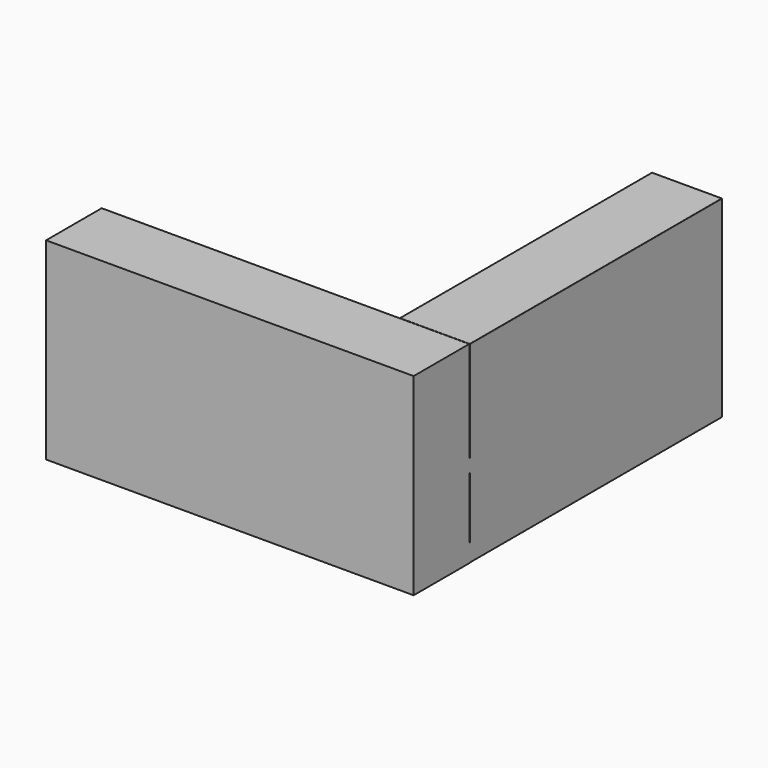
from build123d import *

# Parameters (mm, degrees)
F1_DEPTH = 1800
F3_DEPTH = 1800
F4_DEPTH = 1800
F6_DEPTH = 2100


with BuildPart() as f1:
    # F0 (on Front) → F1 (new body)
    with BuildSketch(Plane.XZ):
        Polygon((-500, 0), (0, -450), (0, -347.4833847613), (-386.0926497348, 0), align=None)
        with BuildLine():
            Line((399, 650), (1, 650))
            ThreePointArc((1, 650), (0.2928932188, 649.7071067812), (0, 649))
            Line((0, 649), (0, 76.2))
            Line((0, 76.2), (-499, 76.2))
            ThreePointArc((-499, 76.2), (-499.7071067812, 75.9071067812), (-500, 75.2))
            Line((-500, 75.2), (-500, 0))
            Line((-500, 0), (-386.0926497348, 0))
            Line((-386.0926497348, 0), (0, 0))
            Line((0, 0), (0, -347.4833847613))
            Line((0, -347.4833847613), (0, -450))
            Line((0, -450), (399, -450))
            ThreePointArc((399, -450), (399.7071067812, -449.7071067812), (400, -449))
            Line((400, -449), (400, 649))
            ThreePointArc((400, 649), (399.7071067812, 649.7071067812), (399, 650))
        make_face()
    extrude(amount=F1_DEPTH)

    # F5 (on offset) → F6 (join)
    with BuildSketch(Plane.YZ.offset(400)):
        with BuildLine():
            ThreePointArc((-1746.6506394539, 125.3499486691), (-1749.4861553685, 124.175439521), (-1750.6606645166, 121.3399236065))
            Line((-1750.6606645166, 121.3399236065), (-1750.6606645166, 81.2396729799))
            ThreePointArc((-1750.6606645166, 81.2396729799), (-1749.4861553685, 78.4041570654), (-1746.6506394539, 77.2296479173))
            Line((-1746.6506394539, 77.2296479173), (-1706.5503888274, 77.2296479173))
            ThreePointArc((-1706.5503888274, 77.2296479173), (-1703.7148729128, 78.4041570654), (-1702.5403637647, 81.2396729799))
            Line((-1702.5403637647, 81.2396729799), (-1702.5403637647, 121.3399236065))
            ThreePointArc((-1702.5403637647, 121.3399236065), (-1703.7148729128, 124.175439521), (-1706.5503888274, 125.3499486691))
            Line((-1706.5503888274, 125.3499486691), (-1746.6506394539, 125.3499486691))
        make_face()
        with BuildLine():
            ThreePointArc((-1752.6656770479, 121.3399236065), (-1753.840186196, 124.175439521), (-1756.6757021106, 125.3499486691))
            Line((-1756.6757021106, 125.3499486691), (-1796.7759527371, 125.3499486691))
            ThreePointArc((-1796.7759527371, 125.3499486691), (-1799.6114686517, 124.175439521), (-1800.7859777998, 121.3399236065))
            Line((-1800.7859777998, 121.3399236065), (-1800.7859777998, 81.2396729799))
            ThreePointArc((-1800.7859777998, 81.2396729799), (-1799.6114686517, 78.4041570654), (-1796.7759527371, 77.2296479173))
            Line((-1796.7759527371, 77.2296479173), (-1756.6757021106, 77.2296479173))
            ThreePointArc((-1756.6757021106, 77.2296479173), (-1753.840186196, 78.4041570654), (-1752.6656770479, 81.2396729799))
            Line((-1752.6656770479, 81.2396729799), (-1752.6656770479, 121.3399236065))
        make_face()
        with BuildLine():
            Line((-1752.6656770479, 131.3649862631), (-1752.6656770479, 171.4652368897))
            ThreePointArc((-1752.6656770479, 171.4652368897), (-1753.840186196, 174.3007528042), (-1756.6757021106, 175.4752619523))
            Line((-1756.6757021106, 175.4752619523), (-1796.7759527371, 175.4752619523))
            ThreePointArc((-1796.7759527371, 175.4752619523), (-1799.6114686517, 174.3007528042), (-1800.7859777998, 171.4652368897))
            Line((-1800.7859777998, 171.4652368897), (-1800.7859777998, 131.3649862631))
            ThreePointArc((-1800.7859777998, 131.3649862631), (-1799.6114686517, 128.5294703486), (-1796.7759527371, 127.3549612005))
            Line((-1796.7759527371, 127.3549612005), (-1756.6757021106, 127.3549612005))
            ThreePointArc((-1756.6757021106, 127.3549612005), (-1753.840186196, 128.5294703486), (-1752.6656770479, 131.3649862631))
        make_face()
        with BuildLine():
            ThreePointArc((-1756.6757021106, 177.4802744837), (-1753.840186196, 178.6547836318), (-1752.6656770479, 181.4902995463))
            Line((-1752.6656770479, 181.4902995463), (-1752.6656770479, 221.5905501729))
            ThreePointArc((-1752.6656770479, 221.5905501729), (-1753.840186196, 224.4260660874), (-1756.6757021106, 225.6005752356))
            Line((-1756.6757021106, 225.6005752356), (-1796.7759527371, 225.6005752356))
            ThreePointArc((-1796.7759527371, 225.6005752356), (-1799.6114686517, 224.4260660874), (-1800.7859777998, 221.5905501729))
            Line((-1800.7859777998, 221.5905501729), (-1800.7859777998, 181.4902995463))
            ThreePointArc((-1800.7859777998, 181.4902995463), (-1799.6114686517, 178.6547836318), (-1796.7759527371, 177.4802744837))
            Line((-1796.7759527371, 177.4802744837), (-1756.6757021106, 177.4802744837))
        make_face()
        with BuildLine():
            ThreePointArc((-1752.6656770479, 422.0918033057), (-1753.840186196, 424.9273192203), (-1756.6757021106, 426.1018283684))
            Line((-1756.6757021106, 426.1018283684), (-1796.7759527371, 426.1018283684))
            ThreePointArc((-1796.7759527371, 426.1018283684), (-1799.6114686517, 424.9273192203), (-1800.7859777998, 422.0918033057))
            Line((-1800.7859777998, 422.0918033057), (-1800.7859777998, 381.9915526792))
            ThreePointArc((-1800.7859777998, 381.9915526792), (-1799.6114686517, 379.1560367646), (-1796.7759527371, 377.9815276165))
            Line((-1796.7759527371, 377.9815276165), (-1756.6757021106, 377.9815276165))
            ThreePointArc((-1756.6757021106, 377.9815276165), (-1753.840186196, 379.1560367646), (-1752.6656770479, 381.9915526792))
            Line((-1752.6656770479, 381.9915526792), (-1752.6656770479, 422.0918033057))
        make_face()
        with BuildLine():
            ThreePointArc((-1800.7859777998, 482.2421792456), (-1799.6114686517, 479.406663331), (-1796.7759527371, 478.2321541829))
            Line((-1796.7759527371, 478.2321541829), (-1756.6757021106, 478.2321541829))
            ThreePointArc((-1756.6757021106, 478.2321541829), (-1753.840186196, 479.406663331), (-1752.6656770479, 482.2421792456))
            Line((-1752.6656770479, 482.2421792456), (-1752.6656770479, 522.3424298721))
            ThreePointArc((-1752.6656770479, 522.3424298721), (-1753.840186196, 525.1779457867), (-1756.6757021106, 526.3524549348))
            Line((-1756.6757021106, 526.3524549348), (-1796.7759527371, 526.3524549348))
            ThreePointArc((-1796.7759527371, 526.3524549348), (-1799.6114686517, 525.1779457867), (-1800.7859777998, 522.3424298721))
            Line((-1800.7859777998, 522.3424298721), (-1800.7859777998, 482.2421792456))
        make_face()
        with BuildLine():
            Line((-1756.6757021106, 476.2271416516), (-1796.7759527371, 476.2271416516))
            ThreePointArc((-1796.7759527371, 476.2271416516), (-1799.6114686517, 475.0526325035), (-1800.7859777998, 472.2171165889))
            Line((-1800.7859777998, 472.2171165889), (-1800.7859777998, 432.1168659624))
            ThreePointArc((-1800.7859777998, 432.1168659624), (-1799.6114686517, 429.2813500478), (-1796.7759527371, 428.1068408997))
            Line((-1796.7759527371, 428.1068408997), (-1756.6757021106, 428.1068408997))
            ThreePointArc((-1756.6757021106, 428.1068408997), (-1753.840186196, 429.2813500478), (-1752.6656770479, 432.1168659624))
            Line((-1752.6656770479, 432.1168659624), (-1752.6656770479, 472.2171165889))
            ThreePointArc((-1752.6656770479, 472.2171165889), (-1753.840186196, 475.0526325035), (-1756.6757021106, 476.2271416516))
        make_face()
        with BuildLine():
            ThreePointArc((-1546.1493863211, 125.3499486691), (-1548.9849022356, 124.175439521), (-1550.1594113838, 121.3399236065))
            Line((-1550.1594113838, 121.3399236065), (-1550.1594113838, 81.2396729799))
            ThreePointArc((-1550.1594113838, 81.2396729799), (-1548.9849022356, 78.4041570654), (-1546.1493863211, 77.2296479173))
            Line((-1546.1493863211, 77.2296479173), (-1506.0491356945, 77.2296479173))
            ThreePointArc((-1506.0491356945, 77.2296479173), (-1503.21361978, 78.4041570654), (-1502.0391106319, 81.2396729799))
            Line((-1502.0391106319, 81.2396729799), (-1502.0391106319, 121.3399236065))
            ThreePointArc((-1502.0391106319, 121.3399236065), (-1503.21361978, 124.175439521), (-1506.0491356945, 125.3499486691))
            Line((-1506.0491356945, 125.3499486691), (-1546.1493863211, 125.3499486691))
        make_face()
        with BuildLine():
            ThreePointArc((-1345.6481331883, 125.3499486691), (-1348.4836491028, 124.175439521), (-1349.6581582509, 121.3399236065))
            Line((-1349.6581582509, 121.3399236065), (-1349.6581582509, 81.2396729799))
            ThreePointArc((-1349.6581582509, 81.2396729799), (-1348.4836491028, 78.4041570654), (-1345.6481331883, 77.2296479173))
            Line((-1345.6481331883, 77.2296479173), (-1305.5478825617, 77.2296479173))
            ThreePointArc((-1305.5478825617, 77.2296479173), (-1302.7123666472, 78.4041570654), (-1301.537857499, 81.2396729799))
            Line((-1301.537857499, 81.2396729799), (-1301.537857499, 121.3399236065))
            ThreePointArc((-1301.537857499, 121.3399236065), (-1302.7123666472, 124.175439521), (-1305.5478825617, 125.3499486691))
            Line((-1305.5478825617, 125.3499486691), (-1345.6481331883, 125.3499486691))
        make_face()
        with BuildLine():
            ThreePointArc((-1445.8987597547, 125.3499486691), (-1448.7342756692, 124.175439521), (-1449.9087848173, 121.3399236065))
            Line((-1449.9087848173, 121.3399236065), (-1449.9087848173, 81.2396729799))
            ThreePointArc((-1449.9087848173, 81.2396729799), (-1448.7342756692, 78.4041570654), (-1445.8987597547, 77.2296479173))
            Line((-1445.8987597547, 77.2296479173), (-1405.7985091281, 77.2296479173))
            ThreePointArc((-1405.7985091281, 77.2296479173), (-1402.9629932136, 78.4041570654), (-1401.7884840655, 81.2396729799))
            Line((-1401.7884840655, 81.2396729799), (-1401.7884840655, 121.3399236065))
            ThreePointArc((-1401.7884840655, 121.3399236065), (-1402.9629932136, 124.175439521), (-1405.7985091281, 125.3499486691))
            Line((-1405.7985091281, 125.3499486691), (-1445.8987597547, 125.3499486691))
        make_face()
        with BuildLine():
            ThreePointArc((-1646.4000128875, 125.3499486691), (-1649.235528802, 124.175439521), (-1650.4100379502, 121.3399236065))
            Line((-1650.4100379502, 121.3399236065), (-1650.4100379502, 81.2396729799))
            ThreePointArc((-1650.4100379502, 81.2396729799), (-1649.235528802, 78.4041570654), (-1646.4000128875, 77.2296479173))
            Line((-1646.4000128875, 77.2296479173), (-1606.2997622609, 77.2296479173))
            ThreePointArc((-1606.2997622609, 77.2296479173), (-1603.4642463464, 78.4041570654), (-1602.2897371983, 81.2396729799))
            Line((-1602.2897371983, 81.2396729799), (-1602.2897371983, 121.3399236065))
            ThreePointArc((-1602.2897371983, 121.3399236065), (-1603.4642463464, 124.175439521), (-1606.2997622609, 125.3499486691))
            Line((-1606.2997622609, 125.3499486691), (-1646.4000128875, 125.3499486691))
        make_face()
        with BuildLine():
            ThreePointArc((-1796.7759527371, 325.851201802), (-1799.6114686517, 324.6766926538), (-1800.7859777998, 321.8411767393))
            Line((-1800.7859777998, 321.8411767393), (-1800.7859777998, 281.7409261127))
            ThreePointArc((-1800.7859777998, 281.7409261127), (-1799.6114686517, 278.9054101982), (-1796.7759527371, 277.7309010501))
            Line((-1796.7759527371, 277.7309010501), (-1756.6757021106, 277.7309010501))
            ThreePointArc((-1756.6757021106, 277.7309010501), (-1753.840186196, 278.9054101982), (-1752.6656770479, 281.7409261127))
            Line((-1752.6656770479, 281.7409261127), (-1752.6656770479, 321.8411767393))
            ThreePointArc((-1752.6656770479, 321.8411767393), (-1753.840186196, 324.6766926538), (-1756.6757021106, 325.851201802))
            Line((-1756.6757021106, 325.851201802), (-1796.7759527371, 325.851201802))
        make_face()
        with BuildLine():
            Line((-1351.6631707822, 81.2396729799), (-1351.6631707822, 121.3399236065))
            ThreePointArc((-1351.6631707822, 121.3399236065), (-1352.8376799304, 124.175439521), (-1355.6731958449, 125.3499486691))
            Line((-1355.6731958449, 125.3499486691), (-1395.7734464715, 125.3499486691))
            ThreePointArc((-1395.7734464715, 125.3499486691), (-1398.608962386, 124.175439521), (-1399.7834715341, 121.3399236065))
            Line((-1399.7834715341, 121.3399236065), (-1399.7834715341, 81.2396729799))
            ThreePointArc((-1399.7834715341, 81.2396729799), (-1398.608962386, 78.4041570654), (-1395.7734464715, 77.2296479173))
            Line((-1395.7734464715, 77.2296479173), (-1355.6731958449, 77.2296479173))
            ThreePointArc((-1355.6731958449, 77.2296479173), (-1352.8376799304, 78.4041570654), (-1351.6631707822, 81.2396729799))
        make_face()
        with BuildLine():
            ThreePointArc((-1455.9238224113, 77.2296479173), (-1453.0883064968, 78.4041570654), (-1451.9137973487, 81.2396729799))
            Line((-1451.9137973487, 81.2396729799), (-1451.9137973487, 121.3399236065))
            ThreePointArc((-1451.9137973487, 121.3399236065), (-1453.0883064968, 124.175439521), (-1455.9238224113, 125.3499486691))
            Line((-1455.9238224113, 125.3499486691), (-1496.0240730379, 125.3499486691))
            ThreePointArc((-1496.0240730379, 125.3499486691), (-1498.8595889524, 124.175439521), (-1500.0340981005, 121.3399236065))
            Line((-1500.0340981005, 121.3399236065), (-1500.0340981005, 81.2396729799))
            ThreePointArc((-1500.0340981005, 81.2396729799), (-1498.8595889524, 78.4041570654), (-1496.0240730379, 77.2296479173))
            Line((-1496.0240730379, 77.2296479173), (-1455.9238224113, 77.2296479173))
        make_face()
        with BuildLine():
            ThreePointArc((-1596.2746996043, 125.3499486691), (-1599.1102155188, 124.175439521), (-1600.284724667, 121.3399236065))
            Line((-1600.284724667, 121.3399236065), (-1600.284724667, 81.2396729799))
            ThreePointArc((-1600.284724667, 81.2396729799), (-1599.1102155188, 78.4041570654), (-1596.2746996043, 77.2296479173))
            Line((-1596.2746996043, 77.2296479173), (-1556.1744489777, 77.2296479173))
            ThreePointArc((-1556.1744489777, 77.2296479173), (-1553.3389330632, 78.4041570654), (-1552.1644239151, 81.2396729799))
            Line((-1552.1644239151, 81.2396729799), (-1552.1644239151, 121.3399236065))
            ThreePointArc((-1552.1644239151, 121.3399236065), (-1553.3389330632, 124.175439521), (-1556.1744489777, 125.3499486691))
            Line((-1556.1744489777, 125.3499486691), (-1596.2746996043, 125.3499486691))
        make_face()
        with BuildLine():
            ThreePointArc((-1696.5253261707, 125.3499486691), (-1699.3608420853, 124.175439521), (-1700.5353512334, 121.3399236065))
            Line((-1700.5353512334, 121.3399236065), (-1700.5353512334, 81.2396729799))
            ThreePointArc((-1700.5353512334, 81.2396729799), (-1699.3608420853, 78.4041570654), (-1696.5253261707, 77.2296479173))
            Line((-1696.5253261707, 77.2296479173), (-1656.4250755442, 77.2296479173))
            ThreePointArc((-1656.4250755442, 77.2296479173), (-1653.5895596296, 78.4041570654), (-1652.4150504815, 81.2396729799))
            Line((-1652.4150504815, 81.2396729799), (-1652.4150504815, 121.3399236065))
            ThreePointArc((-1652.4150504815, 121.3399236065), (-1653.5895596296, 124.175439521), (-1656.4250755442, 125.3499486691))
            Line((-1656.4250755442, 125.3499486691), (-1696.5253261707, 125.3499486691))
        make_face()
        with BuildLine():
            ThreePointArc((-1796.7759527371, 375.9765150852), (-1799.6114686517, 374.8020059371), (-1800.7859777998, 371.9664900225))
            Line((-1800.7859777998, 371.9664900225), (-1800.7859777998, 331.866239396))
            ThreePointArc((-1800.7859777998, 331.866239396), (-1799.6114686517, 329.0307234814), (-1796.7759527371, 327.8562143333))
            Line((-1796.7759527371, 327.8562143333), (-1756.6757021106, 327.8562143333))
            ThreePointArc((-1756.6757021106, 327.8562143333), (-1753.840186196, 329.0307234814), (-1752.6656770479, 331.866239396))
            Line((-1752.6656770479, 331.866239396), (-1752.6656770479, 371.9664900225))
            ThreePointArc((-1752.6656770479, 371.9664900225), (-1753.840186196, 374.8020059371), (-1756.6757021106, 375.9765150852))
            Line((-1756.6757021106, 375.9765150852), (-1796.7759527371, 375.9765150852))
        make_face()
        with BuildLine():
            Line((-1752.6656770479, 231.6156128295), (-1752.6656770479, 271.7158634561))
            ThreePointArc((-1752.6656770479, 271.7158634561), (-1753.840186196, 274.5513793706), (-1756.6757021106, 275.7258885188))
            Line((-1756.6757021106, 275.7258885188), (-1796.7759527371, 275.7258885188))
            ThreePointArc((-1796.7759527371, 275.7258885188), (-1799.6114686517, 274.5513793706), (-1800.7859777998, 271.7158634561))
            Line((-1800.7859777998, 271.7158634561), (-1800.7859777998, 231.6156128295))
            ThreePointArc((-1800.7859777998, 231.6156128295), (-1799.6114686517, 228.780096915), (-1796.7759527371, 227.6055877669))
            Line((-1796.7759527371, 227.6055877669), (-1756.6757021106, 227.6055877669))
            ThreePointArc((-1756.6757021106, 227.6055877669), (-1753.840186196, 228.780096915), (-1752.6656770479, 231.6156128295))
        make_face()
        with BuildLine():
            ThreePointArc((-1756.6757021106, 528.3574674661), (-1753.840186196, 529.5319766143), (-1752.6656770479, 532.3674925288))
            Line((-1752.6656770479, 532.3674925288), (-1752.6656770479, 572.4677431554))
            ThreePointArc((-1752.6656770479, 572.4677431554), (-1753.840186196, 575.3032590699), (-1756.6757021106, 576.477768218))
            Line((-1756.6757021106, 576.477768218), (-1796.7759527371, 576.477768218))
            ThreePointArc((-1796.7759527371, 576.477768218), (-1799.6114686517, 575.3032590699), (-1800.7859777998, 572.4677431554))
            Line((-1800.7859777998, 572.4677431554), (-1800.7859777998, 532.3674925288))
            ThreePointArc((-1800.7859777998, 532.3674925288), (-1799.6114686517, 529.5319766143), (-1796.7759527371, 528.3574674661))
            Line((-1796.7759527371, 528.3574674661), (-1756.6757021106, 528.3574674661))
        make_face()
        with BuildLine():
            Line((-2201.6232628882, -451.0105543268), (-1801.6232628882, -451.0105543268))
            Line((-1801.6232628882, -451.0105543268), (-1801.6232628882, -348.2370052153))
            Line((-1801.6232628882, -348.2370052153), (-1801.6232628882, 0.1172652221))
            Line((-1801.6232628882, 0.1172652221), (-1414.5629624022, 0.1172652221))
            Line((-1414.5629624022, 0.1172652221), (-1300.3701300561, 0.1172652221))
            Line((-1300.3701300561, 0.1172652221), (-1300.3701300561, 76.5082426657))
            Line((-1300.3701300561, 76.5082426657), (-1801.6232628882, 76.5082426657))
            Line((-1801.6232628882, 76.5082426657), (-1801.6232628882, 647.7463379038))
            ThreePointArc((-1801.6232628882, 647.7463379038), (-1802.7948357635, 650.5747650285), (-1805.6232628882, 651.7463379038))
            Line((-1805.6232628882, 651.7463379038), (-2201.6232628882, 651.7463379038))
            Line((-2201.6232628882, 651.7463379038), (-2201.6232628882, -451.0105543268))
        make_face()
        Polygon((-1801.6232628882, -348.2370052153), (-1801.6232628882, -451.0105543268), (-1300.3701300561, 0.1172652221), (-1414.5629624022, 0.1172652221), align=None)
    extrude(amount=-F6_DEPTH)


with BuildPart() as f3:
    # F0 (on Front) → F3 (new body)
    with BuildSketch(Plane.XZ):
        with BuildLine():
            Line((-450.8351918757, 80.9196017385), (-450.8351918757, 120.9196017385))
            ThreePointArc((-450.8351918757, 120.9196017385), (-452.006764751, 123.7480288632), (-454.8351918757, 124.9196017385))
            Line((-454.8351918757, 124.9196017385), (-494.8351918757, 124.9196017385))
            ThreePointArc((-494.8351918757, 124.9196017385), (-497.6636190004, 123.7480288632), (-498.8351918757, 120.9196017385))
            Line((-498.8351918757, 120.9196017385), (-498.8351918757, 80.9196017385))
            ThreePointArc((-498.8351918757, 80.9196017385), (-497.6636190004, 78.0911746137), (-494.8351918757, 76.9196017385))
            Line((-494.8351918757, 76.9196017385), (-454.8351918757, 76.9196017385))
            ThreePointArc((-454.8351918757, 76.9196017385), (-452.006764751, 78.0911746137), (-450.8351918757, 80.9196017385))
        make_face()
    extrude(amount=F3_DEPTH)


with BuildPart() as f3b:
    # F0 (on Front) → F3, piece 2 (new body)
    with BuildSketch(Plane.XZ):
        with BuildLine():
            Line((-400.8351918757, 80.9196017385), (-400.8351918757, 120.9196017385))
            ThreePointArc((-400.8351918757, 120.9196017385), (-402.006764751, 123.7480288632), (-404.8351918757, 124.9196017385))
            Line((-404.8351918757, 124.9196017385), (-444.8351918757, 124.9196017385))
            ThreePointArc((-444.8351918757, 124.9196017385), (-447.6636190004, 123.7480288632), (-448.8351918757, 120.9196017385))
            Line((-448.8351918757, 120.9196017385), (-448.8351918757, 80.9196017385))
            ThreePointArc((-448.8351918757, 80.9196017385), (-447.6636190004, 78.0911746137), (-444.8351918757, 76.9196017385))
            Line((-444.8351918757, 76.9196017385), (-404.8351918757, 76.9196017385))
            ThreePointArc((-404.8351918757, 76.9196017385), (-402.006764751, 78.0911746137), (-400.8351918757, 80.9196017385))
        make_face()
    extrude(amount=F3_DEPTH)


with BuildPart() as f3c:
    # F0 (on Front) → F3, piece 3 (new body)
    with BuildSketch(Plane.XZ):
        with BuildLine():
            Line((-350.8351918757, 80.9196017385), (-350.8351918757, 120.9196017385))
            ThreePointArc((-350.8351918757, 120.9196017385), (-352.006764751, 123.7480288632), (-354.8351918757, 124.9196017385))
            Line((-354.8351918757, 124.9196017385), (-394.8351918757, 124.9196017385))
            ThreePointArc((-394.8351918757, 124.9196017385), (-397.6636190004, 123.7480288632), (-398.8351918757, 120.9196017385))
            Line((-398.8351918757, 120.9196017385), (-398.8351918757, 80.9196017385))
            ThreePointArc((-398.8351918757, 80.9196017385), (-397.6636190004, 78.0911746137), (-394.8351918757, 76.9196017385))
            Line((-394.8351918757, 76.9196017385), (-354.8351918757, 76.9196017385))
            ThreePointArc((-354.8351918757, 76.9196017385), (-352.006764751, 78.0911746137), (-350.8351918757, 80.9196017385))
        make_face()
    extrude(amount=F3_DEPTH)


with BuildPart() as f3d:
    # F0 (on Front) → F3, piece 4 (new body)
    with BuildSketch(Plane.XZ):
        with BuildLine():
            Line((-300.8351918757, 80.9196017385), (-300.8351918757, 120.9196017385))
            ThreePointArc((-300.8351918757, 120.9196017385), (-302.006764751, 123.7480288632), (-304.8351918757, 124.9196017385))
            Line((-304.8351918757, 124.9196017385), (-344.8351918757, 124.9196017385))
            ThreePointArc((-344.8351918757, 124.9196017385), (-347.6636190004, 123.7480288632), (-348.8351918757, 120.9196017385))
            Line((-348.8351918757, 120.9196017385), (-348.8351918757, 80.9196017385))
            ThreePointArc((-348.8351918757, 80.9196017385), (-347.6636190004, 78.0911746137), (-344.8351918757, 76.9196017385))
            Line((-344.8351918757, 76.9196017385), (-304.8351918757, 76.9196017385))
            ThreePointArc((-304.8351918757, 76.9196017385), (-302.006764751, 78.0911746137), (-300.8351918757, 80.9196017385))
        make_face()
    extrude(amount=F3_DEPTH)


with BuildPart() as f3e:
    # F0 (on Front) → F3, piece 5 (new body)
    with BuildSketch(Plane.XZ):
        with BuildLine():
            Line((-250.8351918757, 80.9196017385), (-250.8351918757, 120.9196017385))
            ThreePointArc((-250.8351918757, 120.9196017385), (-252.006764751, 123.7480288632), (-254.8351918757, 124.9196017385))
            Line((-254.8351918757, 124.9196017385), (-294.8351918757, 124.9196017385))
            ThreePointArc((-294.8351918757, 124.9196017385), (-297.6636190004, 123.7480288632), (-298.8351918757, 120.9196017385))
            Line((-298.8351918757, 120.9196017385), (-298.8351918757, 80.9196017385))
            ThreePointArc((-298.8351918757, 80.9196017385), (-297.6636190004, 78.0911746137), (-294.8351918757, 76.9196017385))
            Line((-294.8351918757, 76.9196017385), (-254.8351918757, 76.9196017385))
            ThreePointArc((-254.8351918757, 76.9196017385), (-252.006764751, 78.0911746137), (-250.8351918757, 80.9196017385))
        make_face()
    extrude(amount=F3_DEPTH)


with BuildPart() as f3f:
    # F0 (on Front) → F3, piece 6 (new body)
    with BuildSketch(Plane.XZ):
        with BuildLine():
            Line((-200.8351918757, 80.9196017385), (-200.8351918757, 120.9196017385))
            ThreePointArc((-200.8351918757, 120.9196017385), (-202.006764751, 123.7480288632), (-204.8351918757, 124.9196017385))
            Line((-204.8351918757, 124.9196017385), (-244.8351918757, 124.9196017385))
            ThreePointArc((-244.8351918757, 124.9196017385), (-247.6636190004, 123.7480288632), (-248.8351918757, 120.9196017385))
            Line((-248.8351918757, 120.9196017385), (-248.8351918757, 80.9196017385))
            ThreePointArc((-248.8351918757, 80.9196017385), (-247.6636190004, 78.0911746137), (-244.8351918757, 76.9196017385))
            Line((-244.8351918757, 76.9196017385), (-204.8351918757, 76.9196017385))
            ThreePointArc((-204.8351918757, 76.9196017385), (-202.006764751, 78.0911746137), (-200.8351918757, 80.9196017385))
        make_face()
    extrude(amount=F3_DEPTH)


with BuildPart() as f3g:
    # F0 (on Front) → F3, piece 7 (new body)
    with BuildSketch(Plane.XZ):
        with BuildLine():
            Line((-150.8351918757, 80.9196017385), (-150.8351918757, 120.9196017385))
            ThreePointArc((-150.8351918757, 120.9196017385), (-152.006764751, 123.7480288632), (-154.8351918757, 124.9196017385))
            Line((-154.8351918757, 124.9196017385), (-194.8351918757, 124.9196017385))
            ThreePointArc((-194.8351918757, 124.9196017385), (-197.6636190004, 123.7480288632), (-198.8351918757, 120.9196017385))
            Line((-198.8351918757, 120.9196017385), (-198.8351918757, 80.9196017385))
            ThreePointArc((-198.8351918757, 80.9196017385), (-197.6636190004, 78.0911746137), (-194.8351918757, 76.9196017385))
            Line((-194.8351918757, 76.9196017385), (-154.8351918757, 76.9196017385))
            ThreePointArc((-154.8351918757, 76.9196017385), (-152.006764751, 78.0911746137), (-150.8351918757, 80.9196017385))
        make_face()
    extrude(amount=F3_DEPTH)


with BuildPart() as f3h:
    # F0 (on Front) → F3, piece 8 (new body)
    with BuildSketch(Plane.XZ):
        with BuildLine():
            Line((-100.8351918757, 80.9196017385), (-100.8351918757, 120.9196017385))
            ThreePointArc((-100.8351918757, 120.9196017385), (-102.006764751, 123.7480288632), (-104.8351918757, 124.9196017385))
            Line((-104.8351918757, 124.9196017385), (-144.8351918757, 124.9196017385))
            ThreePointArc((-144.8351918757, 124.9196017385), (-147.6636190004, 123.7480288632), (-148.8351918757, 120.9196017385))
            Line((-148.8351918757, 120.9196017385), (-148.8351918757, 80.9196017385))
            ThreePointArc((-148.8351918757, 80.9196017385), (-147.6636190004, 78.0911746137), (-144.8351918757, 76.9196017385))
            Line((-144.8351918757, 76.9196017385), (-104.8351918757, 76.9196017385))
            ThreePointArc((-104.8351918757, 76.9196017385), (-102.006764751, 78.0911746137), (-100.8351918757, 80.9196017385))
        make_face()
    extrude(amount=F3_DEPTH)


with BuildPart() as f3i:
    # F0 (on Front) → F3, piece 9 (new body)
    with BuildSketch(Plane.XZ):
        with BuildLine():
            Line((-50.8351918757, 80.9196017385), (-50.8351918757, 120.9196017385))
            ThreePointArc((-50.8351918757, 120.9196017385), (-52.006764751, 123.7480288632), (-54.8351918757, 124.9196017385))
            Line((-54.8351918757, 124.9196017385), (-94.8351918757, 124.9196017385))
            ThreePointArc((-94.8351918757, 124.9196017385), (-97.6636190004, 123.7480288632), (-98.8351918757, 120.9196017385))
            Line((-98.8351918757, 120.9196017385), (-98.8351918757, 80.9196017385))
            ThreePointArc((-98.8351918757, 80.9196017385), (-97.6636190004, 78.0911746137), (-94.8351918757, 76.9196017385))
            Line((-94.8351918757, 76.9196017385), (-54.8351918757, 76.9196017385))
            ThreePointArc((-54.8351918757, 76.9196017385), (-52.006764751, 78.0911746137), (-50.8351918757, 80.9196017385))
        make_face()
    extrude(amount=F3_DEPTH)


with BuildPart() as f3j:
    # F0 (on Front) → F3, piece 10 (new body)
    with BuildSketch(Plane.XZ):
        with BuildLine():
            ThreePointArc((-0.8351918757, 120.9196017385), (-2.006764751, 123.7480288632), (-4.8351918757, 124.9196017385))
            Line((-4.8351918757, 124.9196017385), (-44.8351918757, 124.9196017385))
            ThreePointArc((-44.8351918757, 124.9196017385), (-47.6636190004, 123.7480288632), (-48.8351918757, 120.9196017385))
            Line((-48.8351918757, 120.9196017385), (-48.8351918757, 80.9196017385))
            ThreePointArc((-48.8351918757, 80.9196017385), (-47.6636190004, 78.0911746137), (-44.8351918757, 76.9196017385))
            Line((-44.8351918757, 76.9196017385), (-4.8351918757, 76.9196017385))
            ThreePointArc((-4.8351918757, 76.9196017385), (-2.006764751, 78.0911746137), (-0.8351918757, 80.9196017385))
            Line((-0.8351918757, 80.9196017385), (-0.8351918757, 120.9196017385))
        make_face()
    extrude(amount=F3_DEPTH)


with BuildPart() as f4:
    # F0 (on Front) → F4 (new body)
    with BuildSketch(Plane.XZ):
        with BuildLine():
            ThreePointArc((-0.8351918757, 220.9196017385), (-2.006764751, 223.7480288632), (-4.8351918757, 224.9196017385))
            Line((-4.8351918757, 224.9196017385), (-44.8351918757, 224.9196017385))
            ThreePointArc((-44.8351918757, 224.9196017385), (-47.6636190004, 223.7480288632), (-48.8351918757, 220.9196017385))
            Line((-48.8351918757, 220.9196017385), (-48.8351918757, 180.9196017385))
            ThreePointArc((-48.8351918757, 180.9196017385), (-47.6636190004, 178.0911746137), (-44.8351918757, 176.9196017385))
            Line((-44.8351918757, 176.9196017385), (-4.8351918757, 176.9196017385))
            ThreePointArc((-4.8351918757, 176.9196017385), (-2.006764751, 178.0911746137), (-0.8351918757, 180.9196017385))
            Line((-0.8351918757, 180.9196017385), (-0.8351918757, 220.9196017385))
        make_face()
    extrude(amount=F4_DEPTH)


with BuildPart() as f4b:
    # F0 (on Front) → F4, piece 2 (new body)
    with BuildSketch(Plane.XZ):
        with BuildLine():
            ThreePointArc((-0.8351918757, 270.9196017385), (-2.006764751, 273.7480288632), (-4.8351918757, 274.9196017385))
            Line((-4.8351918757, 274.9196017385), (-44.8351918757, 274.9196017385))
            ThreePointArc((-44.8351918757, 274.9196017385), (-47.6636190004, 273.7480288632), (-48.8351918757, 270.9196017385))
            Line((-48.8351918757, 270.9196017385), (-48.8351918757, 230.9196017385))
            ThreePointArc((-48.8351918757, 230.9196017385), (-47.6636190004, 228.0911746137), (-44.8351918757, 226.9196017385))
            Line((-44.8351918757, 226.9196017385), (-4.8351918757, 226.9196017385))
            ThreePointArc((-4.8351918757, 226.9196017385), (-2.006764751, 228.0911746137), (-0.8351918757, 230.9196017385))
            Line((-0.8351918757, 230.9196017385), (-0.8351918757, 270.9196017385))
        make_face()
    extrude(amount=F4_DEPTH)


with BuildPart() as f4c:
    # F0 (on Front) → F4, piece 3 (new body)
    with BuildSketch(Plane.XZ):
        with BuildLine():
            ThreePointArc((-0.8351918757, 320.9196017385), (-2.006764751, 323.7480288632), (-4.8351918757, 324.9196017385))
            Line((-4.8351918757, 324.9196017385), (-44.8351918757, 324.9196017385))
            ThreePointArc((-44.8351918757, 324.9196017385), (-47.6636190004, 323.7480288632), (-48.8351918757, 320.9196017385))
            Line((-48.8351918757, 320.9196017385), (-48.8351918757, 280.9196017385))
            ThreePointArc((-48.8351918757, 280.9196017385), (-47.6636190004, 278.0911746137), (-44.8351918757, 276.9196017385))
            Line((-44.8351918757, 276.9196017385), (-4.8351918757, 276.9196017385))
            ThreePointArc((-4.8351918757, 276.9196017385), (-2.006764751, 278.0911746137), (-0.8351918757, 280.9196017385))
            Line((-0.8351918757, 280.9196017385), (-0.8351918757, 320.9196017385))
        make_face()
    extrude(amount=F4_DEPTH)


with BuildPart() as f4d:
    # F0 (on Front) → F4, piece 4 (new body)
    with BuildSketch(Plane.XZ):
        with BuildLine():
            ThreePointArc((-0.8351918757, 370.9196017385), (-2.006764751, 373.7480288632), (-4.8351918757, 374.9196017385))
            Line((-4.8351918757, 374.9196017385), (-44.8351918757, 374.9196017385))
            ThreePointArc((-44.8351918757, 374.9196017385), (-47.6636190004, 373.7480288632), (-48.8351918757, 370.9196017385))
            Line((-48.8351918757, 370.9196017385), (-48.8351918757, 330.9196017385))
            ThreePointArc((-48.8351918757, 330.9196017385), (-47.6636190004, 328.0911746137), (-44.8351918757, 326.9196017385))
            Line((-44.8351918757, 326.9196017385), (-4.8351918757, 326.9196017385))
            ThreePointArc((-4.8351918757, 326.9196017385), (-2.006764751, 328.0911746137), (-0.8351918757, 330.9196017385))
            Line((-0.8351918757, 330.9196017385), (-0.8351918757, 370.9196017385))
        make_face()
    extrude(amount=F4_DEPTH)


with BuildPart() as f4e:
    # F0 (on Front) → F4, piece 5 (new body)
    with BuildSketch(Plane.XZ):
        with BuildLine():
            ThreePointArc((-0.8351918757, 420.9196017385), (-2.006764751, 423.7480288632), (-4.8351918757, 424.9196017385))
            Line((-4.8351918757, 424.9196017385), (-44.8351918757, 424.9196017385))
            ThreePointArc((-44.8351918757, 424.9196017385), (-47.6636190004, 423.7480288632), (-48.8351918757, 420.9196017385))
            Line((-48.8351918757, 420.9196017385), (-48.8351918757, 380.9196017385))
            ThreePointArc((-48.8351918757, 380.9196017385), (-47.6636190004, 378.0911746137), (-44.8351918757, 376.9196017385))
            Line((-44.8351918757, 376.9196017385), (-4.8351918757, 376.9196017385))
            ThreePointArc((-4.8351918757, 376.9196017385), (-2.006764751, 378.0911746137), (-0.8351918757, 380.9196017385))
            Line((-0.8351918757, 380.9196017385), (-0.8351918757, 420.9196017385))
        make_face()
    extrude(amount=F4_DEPTH)


with BuildPart() as f4f:
    # F0 (on Front) → F4, piece 6 (new body)
    with BuildSketch(Plane.XZ):
        with BuildLine():
            ThreePointArc((-0.8351918757, 470.9196017385), (-2.006764751, 473.7480288632), (-4.8351918757, 474.9196017385))
            Line((-4.8351918757, 474.9196017385), (-44.8351918757, 474.9196017385))
            ThreePointArc((-44.8351918757, 474.9196017385), (-47.6636190004, 473.7480288632), (-48.8351918757, 470.9196017385))
            Line((-48.8351918757, 470.9196017385), (-48.8351918757, 430.9196017385))
            ThreePointArc((-48.8351918757, 430.9196017385), (-47.6636190004, 428.0911746137), (-44.8351918757, 426.9196017385))
            Line((-44.8351918757, 426.9196017385), (-4.8351918757, 426.9196017385))
            ThreePointArc((-4.8351918757, 426.9196017385), (-2.006764751, 428.0911746137), (-0.8351918757, 430.9196017385))
            Line((-0.8351918757, 430.9196017385), (-0.8351918757, 470.9196017385))
        make_face()
    extrude(amount=F4_DEPTH)


with BuildPart() as f4g:
    # F0 (on Front) → F4, piece 7 (new body)
    with BuildSketch(Plane.XZ):
        with BuildLine():
            ThreePointArc((-0.8351918757, 520.9196017385), (-2.006764751, 523.7480288632), (-4.8351918757, 524.9196017385))
            Line((-4.8351918757, 524.9196017385), (-44.8351918757, 524.9196017385))
            ThreePointArc((-44.8351918757, 524.9196017385), (-47.6636190004, 523.7480288632), (-48.8351918757, 520.9196017385))
            Line((-48.8351918757, 520.9196017385), (-48.8351918757, 480.9196017385))
            ThreePointArc((-48.8351918757, 480.9196017385), (-47.6636190004, 478.0911746137), (-44.8351918757, 476.9196017385))
            Line((-44.8351918757, 476.9196017385), (-4.8351918757, 476.9196017385))
            ThreePointArc((-4.8351918757, 476.9196017385), (-2.006764751, 478.0911746137), (-0.8351918757, 480.9196017385))
            Line((-0.8351918757, 480.9196017385), (-0.8351918757, 520.9196017385))
        make_face()
    extrude(amount=F4_DEPTH)


with BuildPart() as f4h:
    # F0 (on Front) → F4, piece 8 (new body)
    with BuildSketch(Plane.XZ):
        with BuildLine():
            ThreePointArc((-0.8351918757, 570.9196017385), (-2.006764751, 573.7480288632), (-4.8351918757, 574.9196017385))
            Line((-4.8351918757, 574.9196017385), (-44.8351918757, 574.9196017385))
            ThreePointArc((-44.8351918757, 574.9196017385), (-47.6636190004, 573.7480288632), (-48.8351918757, 570.9196017385))
            Line((-48.8351918757, 570.9196017385), (-48.8351918757, 530.9196017385))
            ThreePointArc((-48.8351918757, 530.9196017385), (-47.6636190004, 528.0911746137), (-44.8351918757, 526.9196017385))
            Line((-44.8351918757, 526.9196017385), (-4.8351918757, 526.9196017385))
            ThreePointArc((-4.8351918757, 526.9196017385), (-2.006764751, 528.0911746137), (-0.8351918757, 530.9196017385))
            Line((-0.8351918757, 530.9196017385), (-0.8351918757, 570.9196017385))
        make_face()
    extrude(amount=F4_DEPTH)


with BuildPart() as f4i:
    # F0 (on Front) → F4, piece 9 (new body)
    with BuildSketch(Plane.XZ):
        with BuildLine():
            ThreePointArc((-0.8351918757, 170.9196017385), (-2.006764751, 173.7480288632), (-4.8351918757, 174.9196017385))
            Line((-4.8351918757, 174.9196017385), (-44.8351918757, 174.9196017385))
            ThreePointArc((-44.8351918757, 174.9196017385), (-47.6636190004, 173.7480288632), (-48.8351918757, 170.9196017385))
            Line((-48.8351918757, 170.9196017385), (-48.8351918757, 130.9196017385))
            ThreePointArc((-48.8351918757, 130.9196017385), (-47.6636190004, 128.0911746137), (-44.8351918757, 126.9196017385))
            Line((-44.8351918757, 126.9196017385), (-4.8351918757, 126.9196017385))
            ThreePointArc((-4.8351918757, 126.9196017385), (-2.006764751, 128.0911746137), (-0.8351918757, 130.9196017385))
            Line((-0.8351918757, 130.9196017385), (-0.8351918757, 170.9196017385))
        make_face()
    extrude(amount=F4_DEPTH)


solid = Compound([f1.part, f3.part, f3b.part, f3c.part, f3d.part, f3e.part, f3f.part, f3g.part, f3h.part, f3i.part, f3j.part, f4.part, f4b.part, f4c.part, f4d.part, f4e.part, f4f.part, f4g.part, f4h.part, f4i.part])
